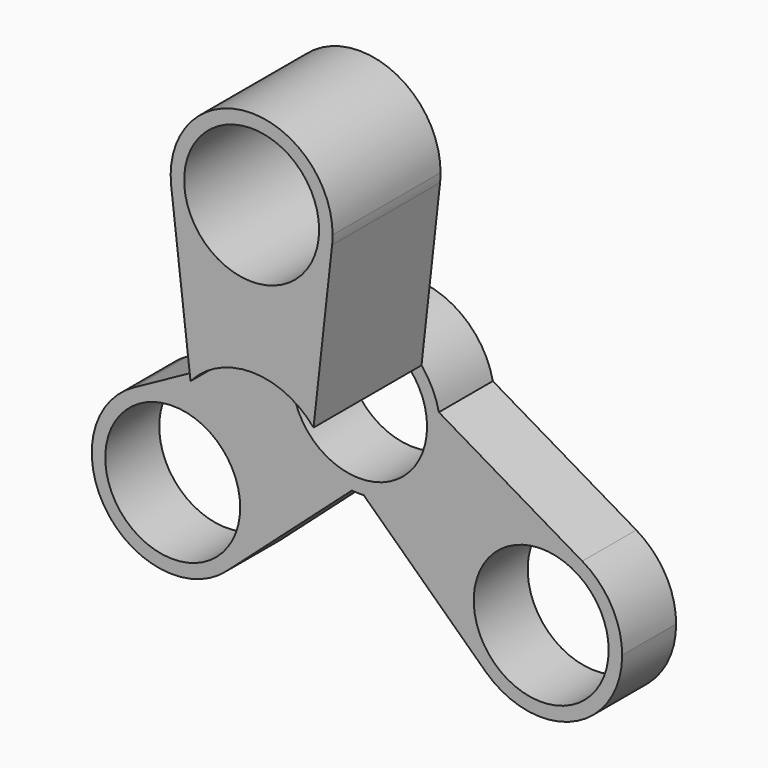
from build123d import *

# Parameters (mm, degrees)
F0_R     = 15.24
F0_R_2   = 12.7
F1_DEPTH = 12.7
F2_R     = 12.7
F3_DEPTH = 25.4
F4_R     = 12.7
F5_DEPTH = 12.7


with BuildPart() as f1:
    # F0 (on Front) → F1 (new body)
    with BuildSketch(Plane.XZ):
        Circle(F0_R)
        Circle(F0_R_2, mode=Mode.SUBTRACT)
    extrude(amount=-F1_DEPTH)

    # F4 (on Front) → F5 (join)
    with BuildSketch(Plane.XZ):
        with BuildLine():
            ThreePointArc((-1.4432226111, -15.1715097632), (-12.4530081547, -8.7852255463), (-14.7768029338, 3.7287658889))
            Line((-14.7768029338, 3.7287658889), (-42.4920327472, -11.4460277555))
            ThreePointArc((-42.4920327472, -11.4460277555), (-27.4039738732, -11.7024445415), (-19.9330004429, -24.813501942))
            ThreePointArc((-19.9330004429, -24.813501942), (-21.266744036, -31.048374254), (-25.0345270501, -36.1919445975))
            Line((-25.0345270501, -36.1919445975), (-1.4432226111, -15.1715097632))
        make_face()
        with BuildLine():
            ThreePointArc((-19.9330004429, -24.813501942), (-27.4039738732, -11.7024445415), (-42.4920327472, -11.4460277555))
            ThreePointArc((-42.4920327472, -11.4460277555), (-47.6260085976, -33.5987274883), (-25.0345270501, -36.1919445975))
            ThreePointArc((-25.0345270501, -36.1919445975), (-21.266744036, -31.048374254), (-19.9330004429, -24.813501942))
        make_face()
        with Locations((-35.1730004429, -24.813501942)):
            Circle(F4_R, mode=Mode.SUBTRACT)
        with BuildLine():
            ThreePointArc((23.6868947427, -36.9702032486), (22.005429254, -16.7439020463), (41.9113655759, -12.7835629617))
            Line((41.9113655759, -12.7835629617), (14.9182126054, 3.11520989))
            ThreePointArc((14.9182126054, 3.11520989), (15.1593396971, 1.5658926996), (15.24, 0))
            ThreePointArc((15.24, 0), (11.0437961568, -10.5020077341), (0.7659624086, -15.2207391932))
            Line((0.7659624086, -15.2207391932), (23.6868947427, -36.9702032486))
        make_face()
        with BuildLine():
            ThreePointArc((23.6868947427, -36.9702032486), (40.1931577089, -39.9173526309), (49.4169899462, -25.9150911903))
            ThreePointArc((49.4169899462, -25.9150911903), (47.4081933041, -18.3524952272), (41.9113655759, -12.7835629617))
            ThreePointArc((41.9113655759, -12.7835629617), (22.005429254, -16.7439020463), (23.6868947427, -36.9702032486))
        make_face()
        with Locations((34.1769899462, -25.9150911903)):
            Circle(F4_R, mode=Mode.SUBTRACT)
    extrude(amount=-F5_DEPTH)


with BuildPart() as f3:
    # F2 (on Front) → F3 (new body)
    with BuildSketch(Plane.XZ):
        with BuildLine():
            ThreePointArc((15.1464025023, 41.2365004611), (0.0390187723, 27.6829937802), (-15.1375684015, 41.1589645532))
            Line((-15.1375684015, 41.1589645532), (-11.5058741435, 9.9936209751))
            ThreePointArc((-11.5058741435, 9.9936209751), (0.1101276854, 15.239602091), (11.649101066, 9.8262935206))
            Line((11.649101066, 9.8262935206), (15.1464025023, 41.2365004611))
        make_face()
        with BuildLine():
            ThreePointArc((15.1464025023, 41.2365004611), (15.2165826343, 42.0784244805), (15.24, 42.9229438305))
            ThreePointArc((15.24, 42.9229438305), (-0.8834753991, 58.13731438), (-15.1375684015, 41.1589645532))
            ThreePointArc((-15.1375684015, 41.1589645532), (0.0390187723, 27.6829937802), (15.1464025023, 41.2365004611))
        make_face()
        with Locations((0, 42.9229438305)):
            Circle(F2_R, mode=Mode.SUBTRACT)
    extrude(amount=F3_DEPTH)


solid = Compound([f1.part, f3.part])
